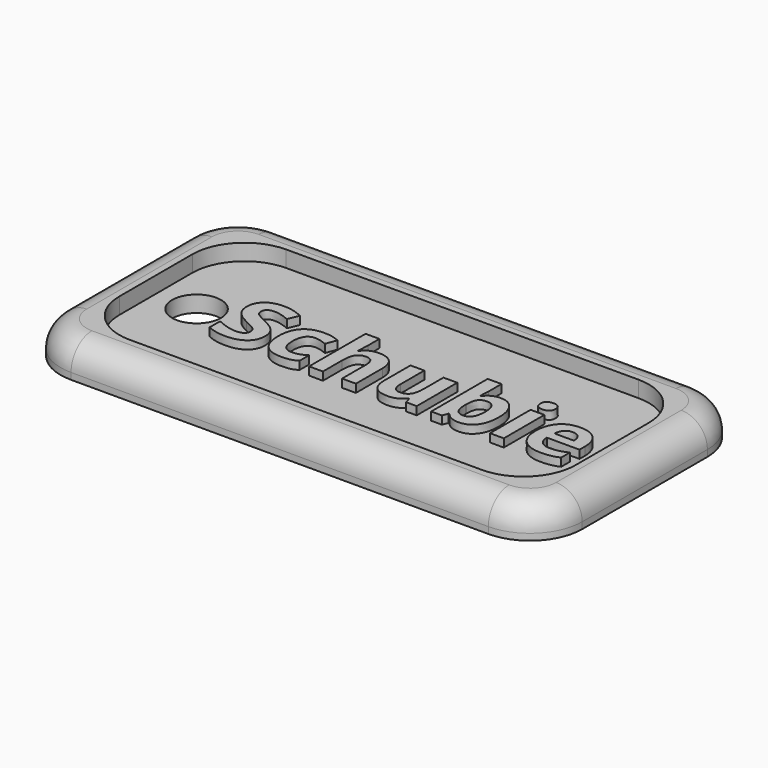
from build123d import *

# Parameters (mm, degrees)
F0_W         = 44.45
F0_H         = 19.05
F0_R         = 2.38125
F1_DEPTH     = 1.5875
F0_W_2       = 50.8
F0_H_2       = 25.4
F2_DEPTH     = 3.175
F3_R         = 5.08
F4_R         = 5.08
F5_TEXT_SIZE = 9.048346056
F6_DEPTH     = 0.79375
F7_R         = 2.54


# Not quite as in the source:
# - a length typed as a fraction of an inch, garbled in the dataset ("3 / 203.2 mm" for 3/8 in), is restored
# - Text() gives the source's letters only with a copy of the font that has no kerning and outlines rounded to 1/6400 em; it was checked with that copy


with BuildPart() as f1:
    # F0 (on Top) → F1 (new body)
    with BuildSketch(Plane.XY):
        with Locations((25.4, 12.7)):
            Rectangle(F0_W, F0_H)
        with Locations((7.14375, 12.7)):
            Circle(F0_R, mode=Mode.SUBTRACT)
    extrude(amount=F1_DEPTH)

    # F0 (on Top) → F2 (join)
    with BuildSketch(Plane.XY):
        with Locations((25.4, 12.7)):
            Rectangle(F0_W_2, F0_H_2)
        with Locations((25.4, 12.7)):
            Rectangle(F0_W, F0_H, mode=Mode.SUBTRACT)
    extrude(amount=F2_DEPTH)

    # F3
    f3_edges = [f1.edges().sort_by_distance(p)[0] for p in [
        (0, 0, 1.5875),
        (50.8, 0, 1.5875),
        (50.8, 25.4, 1.5875),
        (0, 25.4, 1.5875),
    ]]
    fillet(f3_edges, radius=F3_R)

    # F4
    f4_edges = [f1.edges().sort_by_distance(p)[0] for p in [
        (3.175, 22.225, 2.38125),
        (3.175, 3.175, 2.38125),
        (47.625, 3.175, 2.38125),
        (47.625, 22.225, 2.38125),
    ]]
    fillet(f4_edges, radius=F4_R)

    # F5 (on face) → F6 (join)
    with BuildSketch(Plane.XY.offset(1.5875)):
        with Locations((10.3460745861, 9.4682904547)):
            Text('Schubie', F5_TEXT_SIZE, font='Open Sans', font_style=FontStyle.BOLD, text_align=(TextAlign.LEFT, TextAlign.BOTTOM))
    extrude(amount=F6_DEPTH)

    # F7
    f7_edges = [f1.edges().sort_by_distance(p)[0] for p in [
        (25.4, 0, 3.175),
    ]]
    fillet(f7_edges, radius=F7_R)


solid = f1.part
